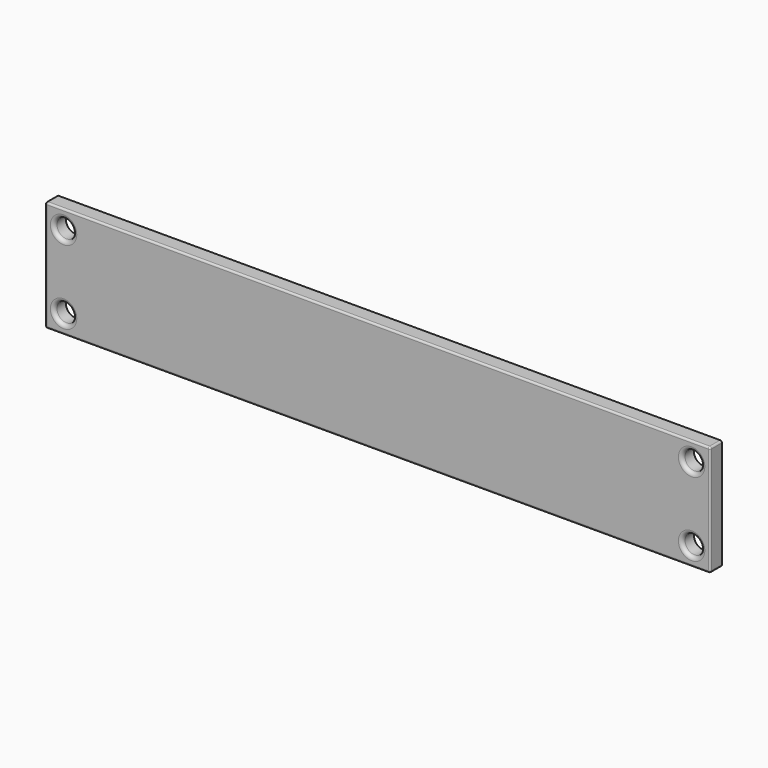
from build123d import *

# Parameters (mm, degrees)
F0_W         = 180
F0_H         = 30
F0_R         = 2.5751263091
F1_DEPTH     = 4
F2_R         = 1
F3_R         = 0.5
F4_TEXT_SIZE = 7.0844787189
F5_DEPTH     = 1


# Not quite as in the source:
# - a feature names something its author has since deleted; it is built from what else it names
# - Text() gives the source's letters only with a copy of the font that has no kerning and outlines rounded to 1/6400 em; it was checked with that copy


with BuildPart() as f1:
    # F0 (on Front) → F1 (new body)
    with BuildSketch(Plane.XZ):
        Rectangle(F0_W, F0_H)
        with Locations((-85, -10)):
            Circle(F0_R, mode=Mode.SUBTRACT)
        with Locations((85, -10)):
            Circle(F0_R, mode=Mode.SUBTRACT)
        with Locations((-85, 10)):
            Circle(F0_R, mode=Mode.SUBTRACT)
        with Locations((85, 10)):
            Circle(F0_R, mode=Mode.SUBTRACT)
    extrude(amount=F1_DEPTH)

    # F2
    f2_edges = [f1.edges().sort_by_distance(p)[0] for p in [
        (-87.575126, -4, 10),
        (-87.575126, -4, -10),
        (82.424874, -4, 10),
        (82.424874, -4, -10),
    ]]
    fillet(f2_edges, radius=F2_R)

    # F3
    f3_edges = [f1.edges().sort_by_distance(p)[0] for p in [
        (0, -4, 15),
        (-90, -4, 0),
        (0, -4, -15),
        (90, -4, 0),
        (-90, -2, 15),
        (-90, -2, -15),
        (90, -2, 15),
        (90, -2, -15),
    ]]
    fillet(f3_edges, radius=F3_R)

    # F4 (on face) → F5 (join)
    with BuildSketch(Plane(origin=(0, 0, 0), x_dir=(-1, 0, 0), z_dir=(0, 1, 0))):
        with Locations((-69.911214523, -1.132793532)):
            Text('New Berea FP Cap', F4_TEXT_SIZE, font='Open Sans', text_align=(TextAlign.LEFT, TextAlign.BOTTOM))
    extrude(amount=F5_DEPTH)

    # F6: F1 across plane


with BuildPart() as f1_1:
    add(f1.part)
    add(f1.part.mirror(Plane.YZ))


solid = f1_1.part
